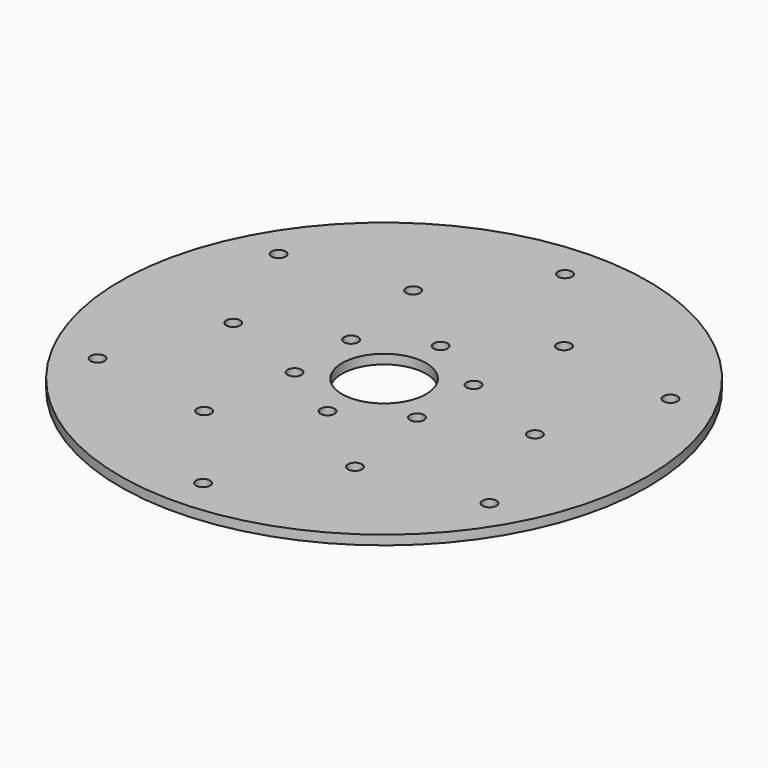
from build123d import *

# Parameters (mm, degrees)
F0_R            = 88.9
F0_R_2          = 14.1605
F1_DEPTH        = 3.175
F2_R            = 2.3622
F3_DEPTH        = 3.176
F3_COPIES_COUNT = 6


# Not quite as in the source:
# - a pattern or mirror of a feature is missing from the dataset's text; its kind, count and spacing are read off the source's solid


with BuildPart() as f1:
    # F0 (on Top) → F1 (new body)
    with BuildSketch(Plane.XY):
        Circle(F0_R)
        Circle(F0_R_2, mode=Mode.SUBTRACT)
    extrude(amount=F1_DEPTH)

    # F2 (on face) → F3 (cut, through all)
    with BuildSketch(Plane.XY.offset(3.175)):
        with Locations((0, 23.8125)):
            Circle(F2_R)
        with Locations((0, 76.2)):
            Circle(F2_R)
        with Locations((25.4, 43.9940905122)):
            Circle(F2_R)
    f3 = extrude(amount=-F3_DEPTH, mode=Mode.SUBTRACT)

    # F3_copies: F3 ×6 about axis
    f3_copies_axis = Axis((0, 0, 0), (0, 0, 1))
    for i in range(1, F3_COPIES_COUNT):
        add(f3.rotate(f3_copies_axis, i * 360 / F3_COPIES_COUNT), mode=Mode.SUBTRACT)


solid = f1.part
